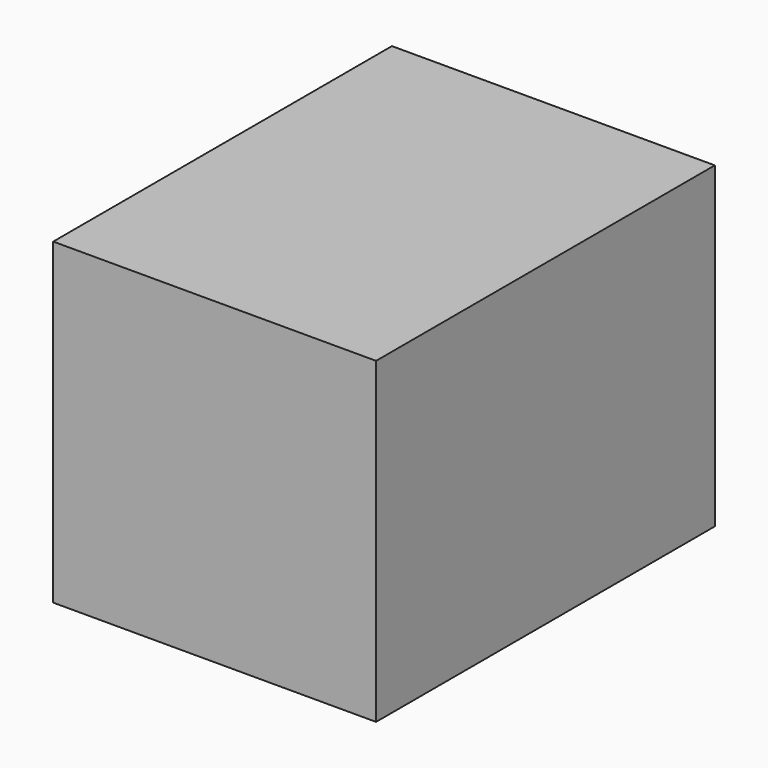
from build123d import *

# Parameters (mm, degrees)
F2_W     = 19.3692743778
F2_H     = 19.0712842159
F3_DEPTH = 25.4


# Not quite as in the source:
# - the program builds the solid bodies; features that only make, move or delete a surface that nothing else refers to are left out


with BuildPart() as f3:
    # F2 (on Front) → F3 (new body)
    with BuildSketch(Plane.XZ):
        with Locations((-9.6846371889, 13.8564801309)):
            Rectangle(F2_W, F2_H)
    extrude(amount=F3_DEPTH)


solid = f3.part
